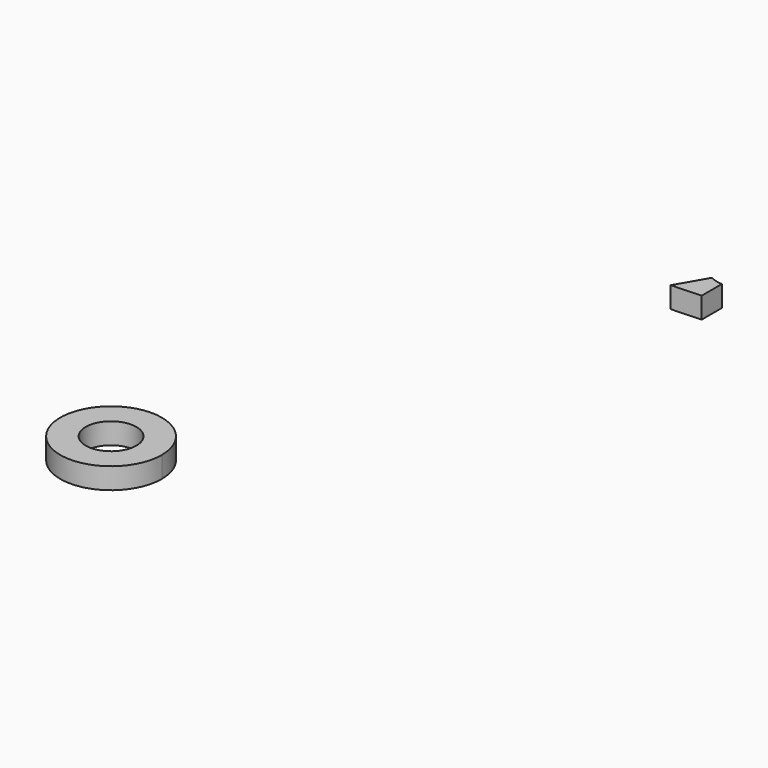
from build123d import *

# Parameters (mm, degrees)
F1_DEPTH = 5
F0_R     = 6


with BuildPart() as f1:
    # F0 (on Top) → F1 (new body)
    with BuildSketch(Plane.XY):
        with BuildLine():
            Line((12.7260516557, 57.8709565262), (8.6399699737, 50.7760246323))
            Line((8.6399699737, 50.7760246323), (15.7204552226, 51.0703360352))
            Line((15.7204552226, 51.0703360352), (15.7204552226, 57.0703360352))
            ThreePointArc((15.7204552226, 57.0703360352), (14.1706612127, 57.2739459063), (12.7260516557, 57.8709565262))
        make_face()
    extrude(amount=F1_DEPTH)


with BuildPart() as f1b:
    # F0 (on Top) → F1, piece 2 (new body)
    with BuildSketch(Plane.XY):
        with BuildLine():
            ThreePointArc((-43.7865273393, -68.3958295986), (-30.4250157042, -72.344591111), (-22.3365694268, -61))
            ThreePointArc((-22.3365694268, -61), (-38.2481231494, -49.655408889), (-43.7865273393, -68.3958295986))
        make_face()
        with Locations((-34.3365694268, -61)):
            Circle(F0_R, mode=Mode.SUBTRACT)
    extrude(amount=F1_DEPTH)


solid = Compound([f1.part, f1b.part])
